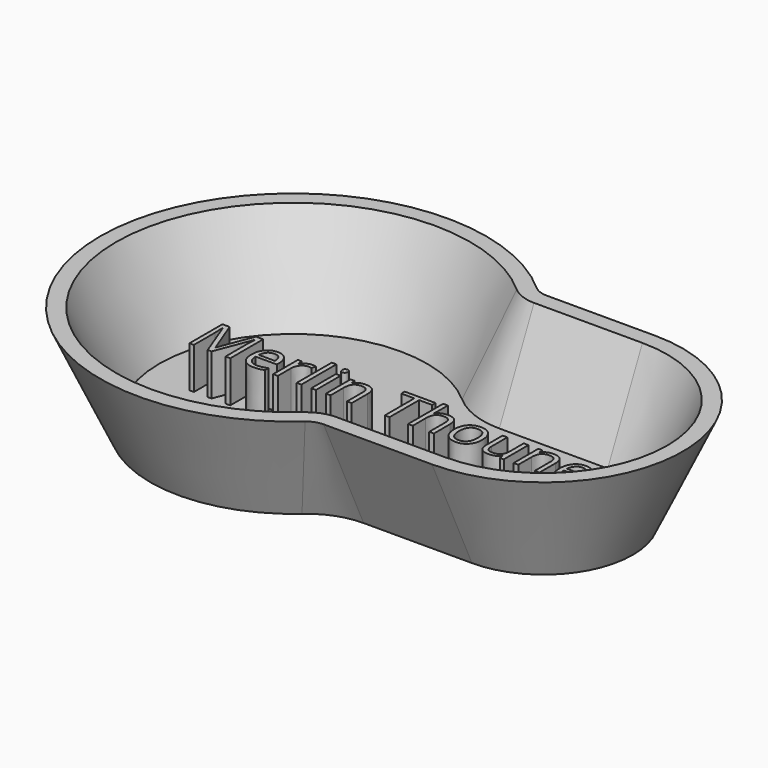
from build123d import *

# Parameters (mm, degrees)
F1_DEPTH     = 15
F1_TAPER     = -25
F2_T         = 2
F3_TEXT_SIZE = 8.0598997092
F4_DEPTH     = 5.8


# Not quite as in the source:
# - a shell that OpenCascade refuses in one call is made with other operations: the cavity is built on its own and cut out
# - Text() gives the source's letters only with a copy of the font that has no kerning and outlines rounded to 1/6400 em; it was checked with that copy


with BuildPart() as f1:
    # F0 (on Top) → F1 (new body)
    with BuildSketch(Plane.XY):
        with BuildLine():
            ThreePointArc((-0.156865167, 12.5), (-3.6923990729, 13.1458565331), (-6.7712434447, 15))
            ThreePointArc((-6.7712434447, 15), (-40, 0), (-6.7712434447, -15))
            ThreePointArc((-6.7712434447, -15), (-3.6923990729, -13.1458565331), (-0.156865167, -12.5))
            Line((-0.156865167, -12.5), (15, -12.5))
            ThreePointArc((15, -12.5), (27.5, 0), (15, 12.5))
            Line((15, 12.5), (-0.156865167, 12.5))
        make_face()
    extrude(amount=F1_DEPTH, taper=F1_TAPER)

    # F2: shell of thickness 2, made by hand


with BuildPart() as f2_core1:
    # F2_t2: copy of F1
    add(f1.part)

    # the walls: a layer under each face that stays
    f2_faces = [f2_core1.faces().sort_by_distance(p)[0] for p in [
        (7.4215674165, 15.9973074362, 7.5),
        (-2.4559141709, 16.4172880836, 7.5),
        (-43.4973074362, 0, 7.5),
        (-2.4559141709, -16.4172880836, 7.5),
        (7.4215674165, -15.9973074362, 7.5),
        (30.9973074362, 0, 7.5),
        (-6.25, 0, 0),
    ]]
    thicken(f2_faces, amount=-F2_T, mode=Mode.SUBTRACT)


with BuildPart() as f1_1:
    add(f1.part)

    # what is left inside the walls is the cavity
    f2_cavity = [f2_core1.part.solids().sort_by_distance(p)[0] for p in [
        (6.595953, 0, 14.98),
    ]]
    add(f2_cavity, mode=Mode.SUBTRACT)

    # F3 (on face) → F4 (join)
    with BuildSketch(Plane.XY.offset(2)):
        with Locations((-33, -2.8690891936)):
            Text('Merlin Thoune', F3_TEXT_SIZE, font='Open Sans', text_align=(TextAlign.LEFT, TextAlign.BOTTOM))
    extrude(amount=F4_DEPTH)


solid = f1_1.part
